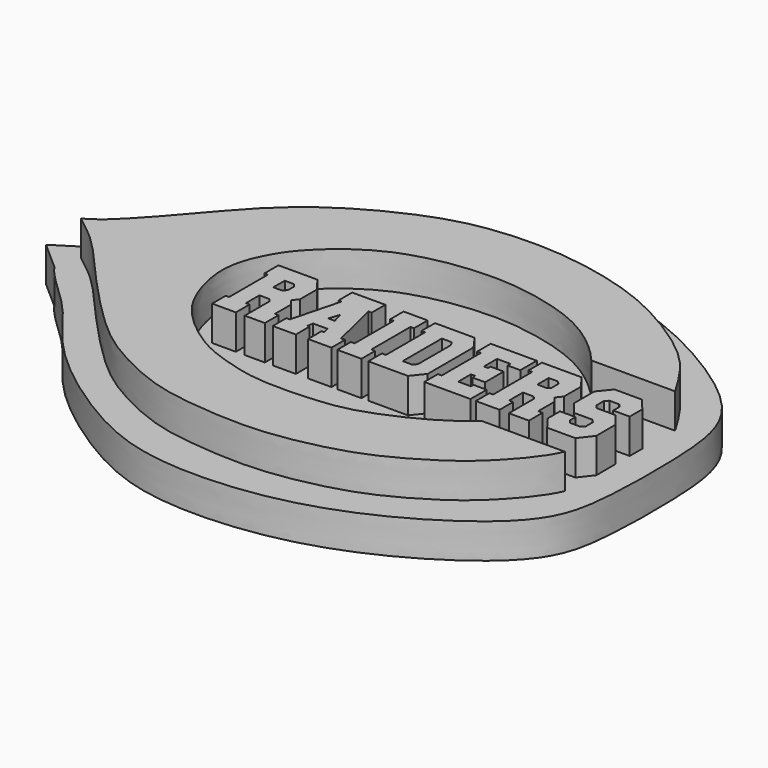
from build123d import *

# Parameters (mm, degrees)
F1_DEPTH     = 6.35
F3_DEPTH     = 6.35
F4_TEXT_SIZE = 5.2916666667
F5_DEPTH     = 3.175


# Not quite as in the source:
# - Text() gives the source's letters only with a copy of the font that has no kerning and outlines rounded to 1/6400 em; it was checked with that copy


with BuildPart() as f1:
    # F0 (on Top) → F1 (new body)
    with BuildSketch(Plane.XY):
        with BuildLine():
            add(Edge.make_bspline(
                [(-57.4096478522, 1.4940799447), (-56.5310329205, 2.0302962099), (-54.2456184789, 3.425078329), (-48.1799133238, 9.9795079324), (-41.92267407, 17.4898285242), (-36.8888128487, 22.6220223599), (-30.2811781752, 27.6627331424), (-21.9646041108, 32.0323569933), (-13.0664974275, 35.3546438999), (-0.70334526, 36.4092337691), (12.0450249548, 34.5976736754), (23.5593988837, 30.5922832843), (34.5380510803, 23.3477595081), (38.988075267, 18.2711717125), (41.1855410102, 14.5899532501), (42.2647818923, 12.7819972113)],
                knots=[0, 0, 0, 0, 0.0477962972, 0.124325622, 0.2057690047, 0.2743106163, 0.3476633892, 0.4261108895, 0.5050358109, 0.5949140278, 0.6868379595, 0.7774724208, 0.8695986004, 0.9359559884, 1, 1, 1, 1], degree=3))
            add(Edge.make_bspline(
                [(-57.4096478522, 1.4940799447), (-56.9156891248, 1.1071363208), (-55.6673626212, 0.1292570876), (-51.7255599336, -2.9447197522), (-46.599651663, -8.9669704184), (-40.8834449932, -15.2348374056), (-35.7355552528, -20.5105873152), (-30.913726946, -24.7913829699), (-25.6198531902, -28.1719650043), (-17.9531637894, -31.7745729651), (-11.0743020063, -33.2426297406), (-1.1440752069, -34.0852940176), (6.7381590783, -33.5811007201), (15.4008508392, -31.7347333026), (22.6658584638, -29.0764738956), (31.544124822, -23.7154162898), (36.3983676265, -19.1544152979), (40.5609458685, -14.1954133287), (41.625842452, -11.6396583617)],
                knots=[0, 0, 0, 0, 0.0333018056, 0.0841599192, 0.1499395163, 0.2179337446, 0.2807593765, 0.3387676112, 0.3969156785, 0.4633871563, 0.5255106422, 0.597752463, 0.6636079104, 0.7312845796, 0.7966034393, 0.8698563963, 0.9309865766, 1, 1, 1, 1], degree=3))
            Line((41.625842452, -11.6396583617), (26.5042968094, -11.6396583617))
            add(Edge.make_bspline(
                [(26.5042968094, -11.6396583617), (24.8554275768, -12.9470878267), (21.1092563228, -15.9175202791), (10.6707832768, -20.6477249304), (3.6619790961, -21.5418089496), (-6.3997098229, -21.9272529677), (-12.9662893286, -20.1856203974), (-18.5117758539, -18.2769608514), (-24.1957845417, -14.3043520227), (-29.2937222605, -9.0396487086), (-31.9054166337, -0.8776997498), (-31.7102046184, 5.264291144), (-28.4173146437, 11.7507036475), (-24.7753582634, 15.5141982447), (-21.02084495, 18.621752308), (-15.8338854397, 21.5930335564), (-8.7295330076, 23.5707653154), (-1.5460390611, 24.2992276205), (5.4272627452, 24.0579892555), (14.6281007291, 21.8816014854), (21.1156117994, 18.5179121358), (25.2974126488, 14.7698074579), (26.9302558154, 12.7819972113)],
                knots=[0, 0, 0, 0, 0.0488582795, 0.1110042438, 0.1617742258, 0.2201009283, 0.2687744913, 0.3132971534, 0.3618662963, 0.412373032, 0.4659353001, 0.512004008, 0.5613663564, 0.6039793591, 0.6445722955, 0.6898714221, 0.7405342597, 0.7903341082, 0.8397670437, 0.8965355789, 0.9473287699, 1, 1, 1, 1], degree=3))
            Line((26.9302558154, 12.7819972113), (42.2647818923, 12.7819972113))
        make_face()
    extrude(amount=F1_DEPTH)



with BuildPart() as f1b:
    # F0 (on Top) → F1, piece 2 (new body)
    with BuildSketch(Plane.XY):
        Polygon((-19.2245659522, 7.8306617215), (-26.3499356806, 7.8306617215), (-26.3499356806, 4.6573723666), (-25.7194824517, 4.6573723666), (-25.7194824517, -4.2320410721), (-26.3499375433, -4.2320410721), (-26.3499375433, -7.3422859423), (-21.9998005778, -7.3422859423), (-21.9998005778, -4.2320410721), (-22.6722843945, -4.2320410721), (-22.6722843945, -1.121798181), (-20.8649821579, -1.121798181), (-20.3816331923, -1.6051467974), (-20.3816331923, -7.3422859423), (-16.7039800435, -7.3422859423), (-16.7039800435, -4.2320410721), (-17.3554494977, -4.2320410721), (-17.3554494977, -0.5754037993), (-18.175041303, 0.4963693791), (-17.3764657229, 1.5681423247), (-17.3764657229, 5.4139168933), align=None)
        Polygon((-20.9933296893, 2.0514912903), (-22.6722843945, 2.0514912903), (-22.6722843945, 4.6783862635), (-20.9700595587, 4.6783862635), (-20.4922624885, 4.0535751305), (-20.4922624885, 2.7239765041), align=None, mode=Mode.SUBTRACT)
    extrude(amount=F1_DEPTH)


with BuildPart() as f1c:
    # F0 (on Top) → F1, piece 3 (new body)
    with BuildSketch(Plane.XY):
        Polygon((-6.7958026193, 7.8306617215), (-12.8582101315, 7.8306617215), (-12.8582101315, 4.7204168513), (-12.2908009216, 4.7204168513), (-14.6234827116, -4.2320410721), (-15.2539378032, -4.2320410721), (-15.2539378032, -7.3422859423), (-11.0298898071, -7.3422859423), (-11.0298898071, -4.2320410721), (-11.4291785285, -4.2320410721), (-11.2190265208, -3.1392534729), (-8.6341612041, -3.1392534729), (-8.3399489522, -4.2320410721), (-8.8022826239, -4.2320410721), (-8.8022826239, -7.3422859423), (-4.5151906088, -7.3422859423), (-4.5151906088, -4.2320410721), (-5.2507212386, -4.2320410721), (-7.3846667074, 4.7204168513), (-6.7958026193, 4.7204168513), align=None)
        Polygon((-9.340537712, -0.5614144611), (-10.5392979458, -0.5614144611), (-9.8673163987, 1.3951907199), align=None, mode=Mode.SUBTRACT)
    extrude(amount=F1_DEPTH)


with BuildPart() as f1d:
    # F0 (on Top) → F1, piece 4 (new body)
    with BuildSketch(Plane.XY):
        Polygon((-2.7578738518, 4.7204168513), (-2.7578738518, -4.2320410721), (-3.4518924076, -4.2320410721), (-3.4518924076, -7.3422859423), (0.9856206598, -7.3422859423), (0.9856206598, -4.2320410721), (0.2916019293, -4.2320410721), (0.2916019293, 4.7204168513), (0.9435581742, 4.7204168513), (0.9435581742, 7.8306617215), (-3.4518924076, 7.8306617215), (-3.4518924076, 4.7204168513), align=None)
    extrude(amount=F1_DEPTH)


with BuildPart() as f1e:
    # F0 (on Top) → F1, piece 5 (new body)
    with BuildSketch(Plane.XY):
        Polygon((9.5306821167, 7.8306617215), (2.2918749601, 7.8306617215), (2.2918749601, 4.7204168513), (2.9636819381, 4.7204168513), (2.9636819381, -4.2320410721), (2.2227098234, -4.2320410721), (2.2227098234, -7.3422859423), (9.4810388982, -7.3422859423), (11.2918764353, -5.0742696039), (11.2918764353, 5.4158177227), align=None)
        Polygon((6.0359546915, -4.2320410721), (6.0359546915, 4.7204168513), (7.8035960905, 4.7204168513), (8.3255339414, 3.962807823), (8.3255339414, -3.6051832139), (7.7360230498, -4.2320410721), align=None, mode=Mode.SUBTRACT)
    extrude(amount=F1_DEPTH)


with BuildPart() as f1f:
    # F0 (on Top) → F1, piece 6 (new body)
    with BuildSketch(Plane.XY):
        Polygon((12.4962273985, 4.7204168513), (13.1695745513, 4.7204168513), (13.1695745513, -4.2320410721), (12.4691594392, -4.2320410721), (12.4691594392, -7.3422859423), (20.9303181618, -7.3422859423), (20.9303181618, -3.6597431172), (18.5311306268, -3.6597431172), (18.5311306268, -4.2320410721), (16.1968041211, -4.2320410721), (16.1968041211, -1.327577047), (16.9960539788, -1.327577047), (16.9960539788, -1.9773773383), (19.3129442632, -1.9773773383), (19.3129442632, 2.2671581246), (16.9137809426, 2.2671581246), (16.9137809426, 1.7198661808), (16.1366723478, 1.7198661808), (16.1366723478, 4.7204168513), (18.5983795673, 4.7204168513), (18.5983795673, 4.0783816949), (20.9149960428, 4.0783816949), (20.9149960428, 7.8306617215), (12.4962273985, 7.8306617215), align=None)
    extrude(amount=F1_DEPTH)


with BuildPart() as f1g:
    # F0 (on Top) → F1, piece 7 (new body)
    with BuildSketch(Plane.XY):
        Polygon((21.860377863, 4.7204168513), (22.5758105516, 4.7204168513), (22.5758105516, -4.2320410721), (21.896449849, -4.2320410721), (21.896449849, -7.3422859423), (26.2539107352, -7.3422859423), (26.2539107352, -4.2320410721), (25.5189947784, -4.2320410721), (25.5189947784, -1.0876338929), (27.4970456958, -1.0876338929), (27.9568396509, -1.6549001448), (27.9568396509, -7.3422859423), (31.6199325025, -7.3422859423), (31.6199325025, -4.2320410721), (30.8221597224, -4.2320410721), (30.8221597224, -0.5614144611), (30.0230123103, 0.5121445283), (30.8672431856, 1.6480567865), (30.8672431856, 5.5371369235), (29.0797632188, 7.8306617215), (21.860377863, 7.8306617215), align=None)
        Polygon((25.584993884, 2.1287021227), (25.584993884, 4.7204168513), (27.3105502129, 4.7204168513), (27.8153009713, 4.1471431032), (27.8153009713, 2.6336531155), (27.4355188012, 2.1287021227), align=None, mode=Mode.SUBTRACT)
    extrude(amount=F1_DEPTH)


with BuildPart() as f1h:
    # F0 (on Top) → F1, piece 8 (new body)
    with BuildSketch(Plane.XY):
        Polygon((40.1905030012, 7.8306617215), (35.1401381195, 7.8306617215), (33.2818776369, 5.5390750058), (33.2818776369, 0.8511532797), (35.1355150342, -1.4358583139), (38.5234542191, -1.4358583139), (39.0726178885, -2.0240072627), (39.0726178885, -3.6660928745), (38.3957996964, -4.2123366147), (36.6492345929, -4.2123366147), (36.1451245844, -3.6660928745), (36.1451245844, -2.3231380619), (33.2818776369, -2.3231380619), (33.2818776369, -5.1401057281), (35.0273549557, -7.4257217348), (40.1905030012, -7.4257217348), (42.083196342, -4.9856323749), (42.0591048896, -0.6130600232), (40.1905030012, 1.7159794224), (36.7363616824, 1.7159794224), (36.1904390156, 2.3882163223), (36.1904390156, 4.1120504029), (36.7588847876, 4.6605649404), (38.526494056, 4.6605649404), (39.0726178885, 4.0934383869), (39.0726178885, 2.6243682951), (42.083196342, 2.6243682951), (42.083196342, 5.5044027977), align=None)
    extrude(amount=F1_DEPTH)


with BuildPart() as f1_1:
    add(f1.part)

    add(f1b.part)  # F3 merges F1b

    add(f1c.part)  # F3 merges F1c

    add(f1d.part)  # F3 merges F1d

    add(f1e.part)  # F3 merges F1e

    add(f1f.part)  # F3 merges F1f

    add(f1g.part)  # F3 merges F1g

    add(f1h.part)  # F3 merges F1h
    # F2 (on face) → F3 (join)
    with BuildSketch(Plane(origin=(0, 0, 0), x_dir=(1, 0, 0), z_dir=(0, 0, -1))):
        with BuildLine():
            add(Edge.make_bspline(
                [(-58.6332827806, 3.0538167339), (-59.689860791, 1.9430531344), (-62.7681948245, -0.4161447675), (-63.8247728348, -1.5269083669)],
                knots=[0, 0, 0, 0, 6.9234826086, 6.9234826086, 6.9234826086, 6.9234826086], degree=3))
            add(Edge.make_bspline(
                [(-63.8247728348, -1.5269083669), (-62.6652246228, -2.4806865024), (-58.5940814135, -4.2779081622), (-51.6439373364, -13.0686686653), (-44.0793115449, -21.5059854404), (-34.0769718857, -30.2306714706), (-22.0518416963, -37.3231662949), (-4.9998142036, -41.965345955), (16.0037934292, -40.4658300055), (35.6731951809, -29.91090589), (46.5600255448, -20.0445269979), (47.9154740285, -6.6812646016), (47.7492442053, 8.7738383331), (46.0345472451, 20.2440011264), (33.0432792391, 31.0162445717), (13.258682741, 40.1753161546), (-9.6395802355, 41.469314141), (-24.5076425254, 36.073659974), (-42.4781037832, 22.9957132986), (-49.2717465337, 11.6411950025), (-56.9433767009, 5.5970726713), (-58.6332827806, 3.0538167339)],
                knots=[0, 0, 0, 0, 0.03192039, 0.0771001544, 0.1235587668, 0.1726321292, 0.2231927225, 0.2796867975, 0.3419557876, 0.4060240908, 0.4564082617, 0.5049654134, 0.5585549254, 0.6034568306, 0.6572652255, 0.7214872158, 0.7853613612, 0.8396362877, 0.9024932481, 0.9531441217, 1, 1, 1, 1], degree=3))
        make_face()
    extrude(amount=F3_DEPTH)

    # F4 (on face) → F5 (cut)
    with BuildSketch(Plane(origin=(0, 0, -6.35), x_dir=(1, 0, 0), z_dir=(0, 0, -1))):
        with Locations(Location((-39.3151826556, 16.3743826647), (0, 0, -140))):
            Text('R. Frisell', F4_TEXT_SIZE, font='Open Sans', font_style=FontStyle.BOLD, text_align=(TextAlign.LEFT, TextAlign.BOTTOM))
    extrude(amount=-F5_DEPTH, mode=Mode.SUBTRACT)


solid = f1_1.part
